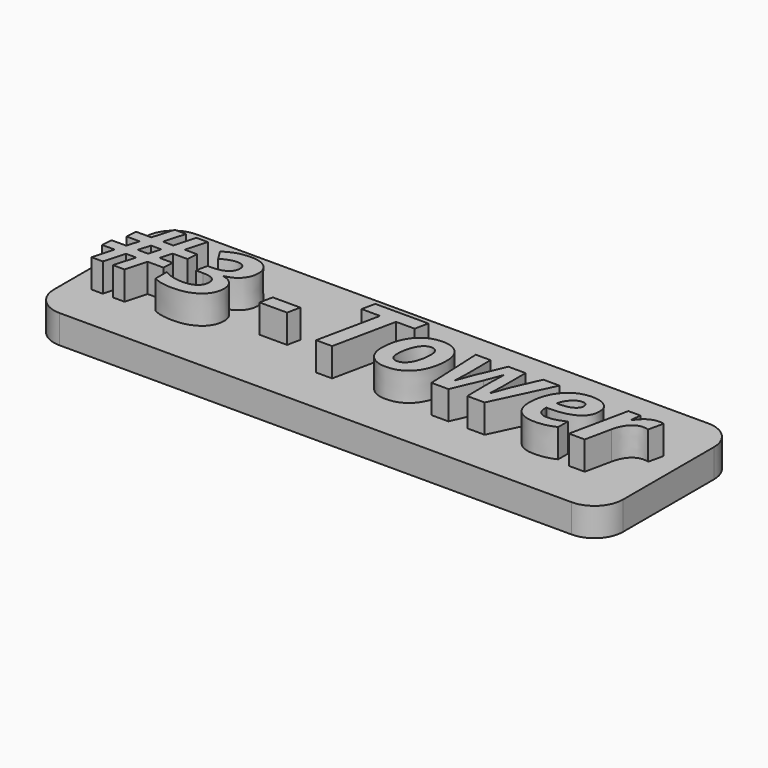
from build123d import *

# Parameters (mm, degrees)
F0_W         = 50.8
F0_H         = 15.24
F1_DEPTH     = 2.54
F2_TEXT_SIZE = 9.6096574469
F3_DEPTH     = 2.54
F4_R         = 2.54


# Not quite as in the source:
# - Text() gives the source's letters only with a copy of the font that has no kerning and outlines rounded to 1/6400 em; it was checked with that copy


with BuildPart() as f1:
    # F0 (on Top) → F1 (new body)
    with BuildSketch(Plane.XY):
        Rectangle(F0_W, F0_H)
    extrude(amount=F1_DEPTH)

    # F2 (on face) → F3 (join)
    with BuildSketch(Plane.XY.offset(2.54)):
        with Locations((-24.13, -3.4594766809)):
            Text('#3 - Tower', F2_TEXT_SIZE, font='Open Sans', font_style=FontStyle.BOLDITALIC, text_align=(TextAlign.LEFT, TextAlign.BOTTOM))
    extrude(amount=F3_DEPTH)

    # F4
    f4_edges = [f1.edges().sort_by_distance(p)[0] for p in [
        (-25.4, 7.62, 1.27),
        (-25.4, -7.62, 1.27),
        (25.4, -7.62, 1.27),
        (25.4, 7.62, 1.27),
    ]]
    fillet(f4_edges, radius=F4_R)


solid = f1.part
